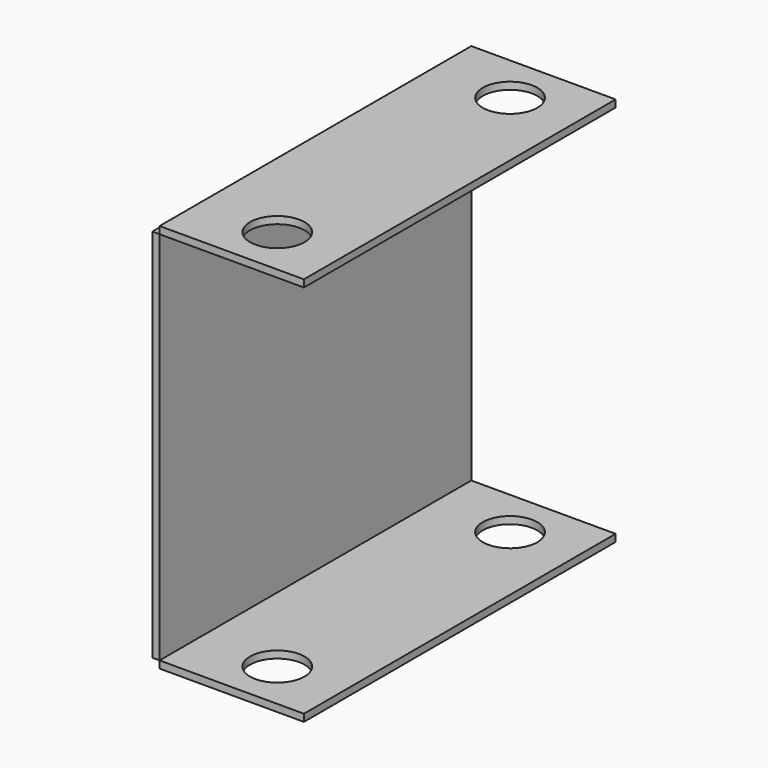
from build123d import *

# Parameters (mm, degrees)
F0_W     = 31.75
F0_H     = 85.725
F0_R     = 5.9944
F1_DEPTH = 1.5875
F0_W_2   = 82.55
F2_DEPTH = 1.5875
F4_ANGLE = 90


# Not quite as in the source:
# - a feature of the source that left no trace in its solid (it failed there, or was rolled back) is left out
# - a pattern or mirror of a feature is missing from the dataset's text; its kind, count and spacing are read off the source's solid


with BuildPart() as f1:
    # F0 (on Top) → F1 (new body)
    with BuildSketch(Plane.XY):
        with Locations((-103.5607946515, 12.7495256543)):
            Rectangle(F0_W, F0_H)
        with Locations((-102.2272946515, -19.2544743457)):
            Circle(F0_R, mode=Mode.SUBTRACT)
        with Locations((-102.2272946515, 44.7535256543)):
            Circle(F0_R, mode=Mode.SUBTRACT)
    extrude(amount=F1_DEPTH)


with BuildPart() as f1_copies_1:
    # F1_copies: instance of F1
    add(f1.part.mirror(Plane(origin=(0, 0, -41.275), x_dir=(-1, 0, 0), z_dir=(0, 0, -1))))


with BuildPart() as f2:
    # F0 (on Top) → F2 (new body)
    with BuildSketch(Plane.XY):
        with Locations((-160.7107946515, 12.7495256543)):
            Rectangle(F0_W_2, F0_H)
    extrude(amount=F2_DEPTH)


with BuildPart() as f2_1:
    # F4: moved
    add(f2.part.rotate(Axis((-119.4357946515, 12.7495256543, 0), (0, -1, 0)), F4_ANGLE))


solid = Compound([f1.part, f1_copies_1.part, f2_1.part])
